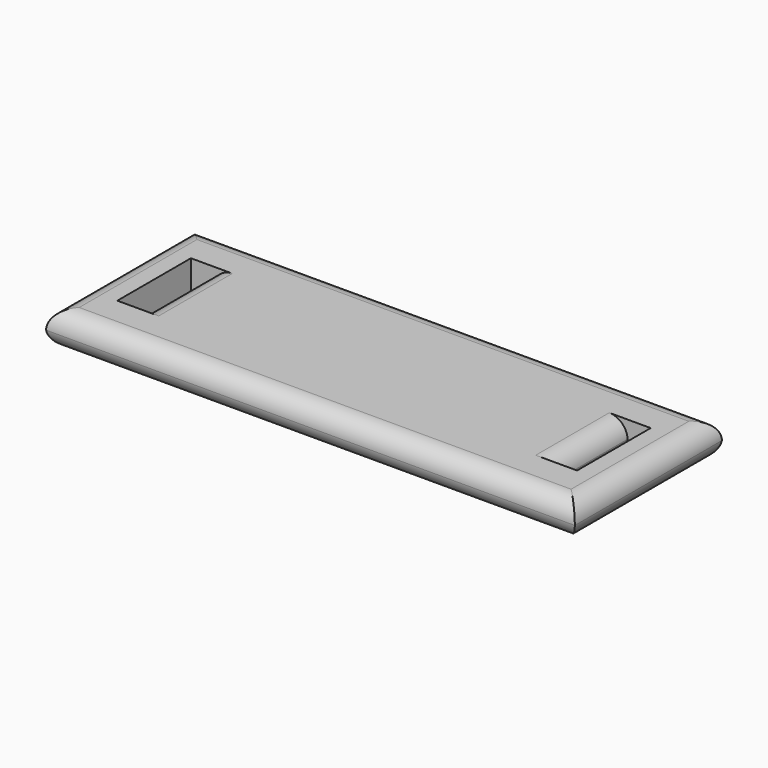
from build123d import *

# Parameters (mm, degrees)
F0_W        = 146.05
F0_H        = 50.8
F0_W_2      = 6.35
F0_H_2      = 25.4
F1_DEPTH    = 9.525
F2_R        = 5.08
F3_T1_DEPTH = 171.2507812379
F3_T3_DEPTH = 76.0007812379
F3_T5_DEPTH = 25.4


# Not quite as in the source:
# - a fillet or chamfer that OpenCascade refuses, or shapes differently, is made with other operations: its cross-section is extruded or revolved along the edge and cut away or added


with BuildPart() as f1:
    # F0 (on Top) → F1 (new body)
    with BuildSketch(Plane.XY):
        Rectangle(F0_W, F0_H)
        with Locations((-60.325, 0)):
            Rectangle(F0_W_2, F0_H_2, mode=Mode.SUBTRACT)
        with Locations((60.325, 0)):
            Rectangle(F0_W_2, F0_H_2, mode=Mode.SUBTRACT)
    extrude(amount=F1_DEPTH)

    # F2
    f2_edges = [f1.edges().sort_by_distance(p)[0] for p in [
        (0, 25.4, 9.525),
        (73.025, 0, 9.525),
        (0, -25.4, 9.525),
        (-73.025, 0, 9.525),
    ]]
    fillet(f2_edges, radius=F2_R)

    # F3: fillet of radius 5.08 on 8 edges, made by hand

    # F3_s2 → F3_t1 (cut)
    with BuildSketch(Plane.YZ.offset(-85.6253906189)):
        with BuildLine():
            ThreePointArc((-25.4, 4.445), (-23.7199479175, 1.27), (-20.3598437524, 0))
            Line((-20.3598437524, 0), (-20.3598437524, -0.1016))
            Line((-20.3598437524, -0.1016), (-25.4, -0.1016))
            Line((-25.4, -0.1016), (-25.5016, 0))
            ThreePointArc((-25.5016, 0), (-25.5016, 2.2225), (-25.500803125, 4.4323))
            Line((-25.500803125, 4.4323), (-25.4, 4.445))
        make_face()
        with BuildLine():
            ThreePointArc((20.3598437524, 0), (23.7199479175, 1.27), (25.4, 4.445))
            Line((25.4, 4.445), (25.500803125, 4.4323))
            ThreePointArc((25.500803125, 4.4323), (25.5016, 2.2225), (25.5016, 0))
            Line((25.5016, 0), (25.4, -0.1016))
            Line((25.4, -0.1016), (20.3598437524, -0.1016))
            Line((20.3598437524, -0.1016), (20.3598437524, 0))
        make_face()
    extrude(amount=F3_T1_DEPTH, mode=Mode.SUBTRACT)

    # F3_s4 → F3_t3 (cut)
    with BuildSketch(Plane.XZ.offset(-38.0003906189)):
        with BuildLine():
            ThreePointArc((-73.025, 4.445), (-71.3449479175, 1.27), (-67.9848437524, 0))
            Line((-67.9848437524, 0), (-67.9848437524, -0.1016))
            Line((-67.9848437524, -0.1016), (-73.025, -0.1016))
            Line((-73.025, -0.1016), (-73.1266, 0))
            ThreePointArc((-73.1266, 0), (-73.1266, 2.2225), (-73.125803125, 4.4323))
            Line((-73.125803125, 4.4323), (-73.025, 4.445))
        make_face()
        with BuildLine():
            ThreePointArc((67.9848437524, 0), (71.3449479175, 1.27), (73.025, 4.445))
            Line((73.025, 4.445), (73.125803125, 4.4323))
            ThreePointArc((73.125803125, 4.4323), (73.1266, 2.2225), (73.1266, 0))
            Line((73.1266, 0), (73.025, -0.1016))
            Line((73.025, -0.1016), (67.9848437524, -0.1016))
            Line((67.9848437524, -0.1016), (67.9848437524, 0))
        make_face()
    extrude(amount=F3_T3_DEPTH, mode=Mode.SUBTRACT)

    # F3_s6 → F3_t5 (cut)
    with BuildSketch(Plane.XZ.offset(-12.7)):
        with BuildLine():
            ThreePointArc((52.07, 9.525), (55.6621024484, 8.0371024484), (57.15, 4.445))
            Line((57.15, 4.445), (57.2516, 4.445))
            Line((57.2516, 4.445), (57.2516, 9.6266))
            Line((57.2516, 9.6266), (52.07, 9.6266))
            Line((52.07, 9.6266), (52.07, 9.525))
        make_face()
        with BuildLine():
            ThreePointArc((52.07, 0), (55.6621024484, 1.4878975516), (57.15, 5.08))
            Line((57.15, 5.08), (57.2516, 5.08))
            Line((57.2516, 5.08), (57.2516, -0.1016))
            Line((57.2516, -0.1016), (52.07, -0.1016))
            Line((52.07, -0.1016), (52.07, 0))
        make_face()
        with BuildLine():
            ThreePointArc((-52.07, 9.525), (-55.6621024484, 8.0371024484), (-57.15, 4.445))
            Line((-57.15, 4.445), (-57.2516, 4.445))
            Line((-57.2516, 4.445), (-57.2516, 9.6266))
            Line((-57.2516, 9.6266), (-52.07, 9.6266))
            Line((-52.07, 9.6266), (-52.07, 9.525))
        make_face()
        with BuildLine():
            ThreePointArc((-52.07, 0), (-55.6621024484, 1.4878975516), (-57.15, 5.08))
            Line((-57.15, 5.08), (-57.2516, 5.08))
            Line((-57.2516, 5.08), (-57.2516, -0.1016))
            Line((-57.2516, -0.1016), (-52.07, -0.1016))
            Line((-52.07, -0.1016), (-52.07, 0))
        make_face()
    extrude(amount=F3_T5_DEPTH, mode=Mode.SUBTRACT)


solid = f1.part
